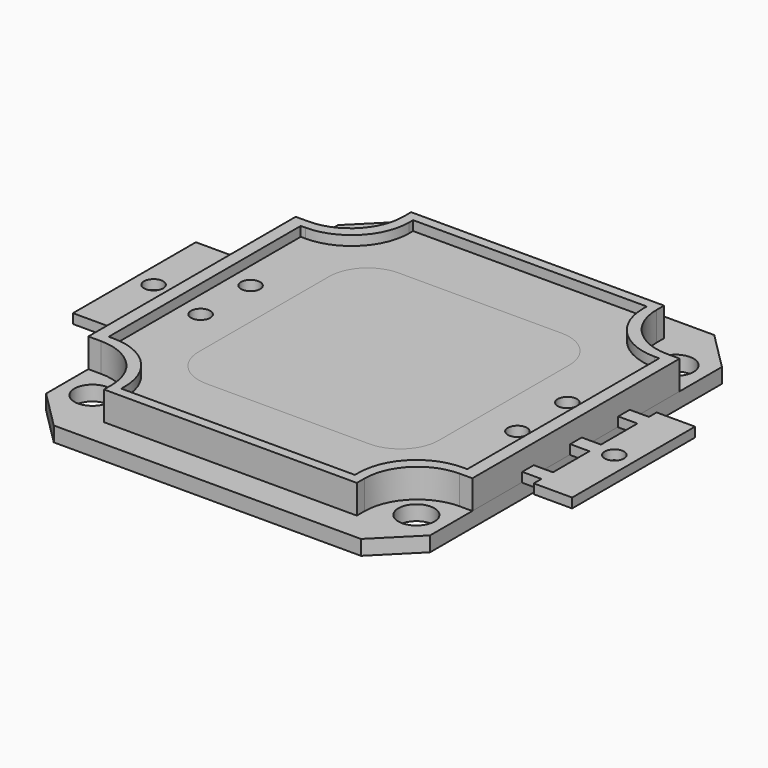
from build123d import *

# Parameters (mm, degrees)
F1_DEPTH = 1.55
F3_SIZE  = 4
F4_R     = 1.875
F5_DEPTH = 4
F6_DEPTH = 3
F2_R     = 1
F2_W     = 1.5
F2_H     = 0.5
F2_W_2   = 0.5
F2_H_2   = 1.5219762474
F2_H_3   = 1.4780237526
F7_DEPTH = 2
F8_DEPTH = 2
F9_START = 1.5
F0_R     = 1
F0_W     = 2
F0_H     = 1.5
F9_DEPTH = 1


with BuildPart() as f1:
    # F0 (on Top) → F1 (new body)
    with BuildSketch(Plane.XY):
        Polygon((20, 23), (-20, 23), (-20, 7), (-20, 5.5), (-20, 0.75), (-20, -0.75), (-20, -5.5), (-20, -7), (-20, -23), (20, -23), (20, -7), (20, -5.5), (20, -0.75), (20, 0.75), (20, 5.5), (20, 7), align=None)
    extrude(amount=F1_DEPTH)

    # F3
    f3_edges = [f1.edges().sort_by_distance(p)[0] for p in [
        (-20, 23, 0.775),
        (20, 23, 0.775),
        (20, -23, 0.775),
        (-20, -23, 0.775),
    ]]
    chamfer(f3_edges, length=F3_SIZE)

    # F4 (on face) → F5 (cut)
    with BuildSketch(Plane.XY.offset(1.55)):
        with Locations((-16.875, -16.875)):
            Circle(F4_R)
        with Locations((16.875, -16.875)):
            Circle(F4_R)
        with Locations((16.875, 16.875)):
            Circle(F4_R)
        with Locations((-16.875, 16.875)):
            Circle(F4_R)
    extrude(amount=-F5_DEPTH, mode=Mode.SUBTRACT)

    # F0 (on Top) → F9 (join)
    with BuildSketch(Plane.XY.offset(F9_START)):
        Polygon((-20, 5.5), (-20, 7), (-22, 7), (-22, 8), (-26, 8), (-26, -8), (-22, -8), (-22, -7), (-20, -7), (-20, -5.5), (-22, -5.5), (-22, -0.75), (-22, 0.75), (-22, 5.5), align=None)
        with Locations((-24, 0)):
            Circle(F0_R, mode=Mode.SUBTRACT)
        Polygon((22, 7), (20, 7), (20, 5.5), (22, 5.5), (22, 0.75), (22, -0.75), (22, -5.5), (20, -5.5), (20, -7), (22, -7), (22, -8), (26, -8), (26, 8), (22, 8), align=None)
        with Locations((24, 0)):
            Circle(F0_R, mode=Mode.SUBTRACT)
        with Locations((21, 0)):
            Rectangle(F0_W, F0_H)
        with Locations((-21, 0)):
            Rectangle(F0_W, F0_H)
    extrude(amount=F9_DEPTH)


with BuildPart() as f6:
    # F2 (on face) → F6 (new body)
    with BuildSketch(Plane.XY.offset(1.55)):
        with BuildLine():
            Line((13.1731458455, 20), (-13.1731458455, 20))
            Line((-13.1731458455, 20), (-13.1731458455, 19))
            ThreePointArc((-13.1731458455, 19), (-14.784058549, 15.1109127035), (-18.6731458455, 13.5))
            Line((-18.6731458455, 13.5), (-20, 13.5))
            Line((-20, 13.5), (-20, -13.5))
            Line((-20, -13.5), (-18.6731458455, -13.5))
            ThreePointArc((-18.6731458455, -13.5), (-14.784058549, -15.1109127035), (-13.1731458455, -19))
            Line((-13.1731458455, -19), (-13.1731458455, -20))
            Line((-13.1731458455, -20), (13.1731458455, -20))
            Line((13.1731458455, -20), (13.1731458455, -19))
            ThreePointArc((13.1731458455, -19), (14.784058549, -15.1109127035), (18.6731458455, -13.5))
            Line((18.6731458455, -13.5), (20, -13.5))
            Line((20, -13.5), (20, 13.5))
            Line((20, 13.5), (18.6731458455, 13.5))
            ThreePointArc((18.6731458455, 13.5), (14.784058549, 15.1109127035), (13.1731458455, 19))
            Line((13.1731458455, 19), (13.1731458455, 20))
        make_face()
        with BuildLine():
            Line((-12.1731458455, 18.5), (-12.1731458455, 19))
            Line((-12.1731458455, 19), (12.1731458455, 19))
            Line((12.1731458455, 19), (12.1731458455, 18.5))
            ThreePointArc((12.1731458455, 18.5), (13.9305051584, 14.2573593129), (18.1731458455, 12.5))
            Line((18.1731458455, 12.5), (18.6731458455, 12.5))
            Line((18.6731458455, 12.5), (18.6731458455, -12.5))
            Line((18.6731458455, -12.5), (18.1731458455, -12.5))
            ThreePointArc((18.1731458455, -12.5), (13.9305051584, -14.2573593129), (12.1731458455, -18.5))
            Line((12.1731458455, -18.5), (12.1731458455, -19))
            Line((12.1731458455, -19), (-12.1731458455, -19))
            Line((-12.1731458455, -19), (-12.1731458455, -18.5))
            ThreePointArc((-12.1731458455, -18.5), (-13.9305051584, -14.2573593129), (-18.1731458455, -12.5))
            Line((-18.1731458455, -12.5), (-18.6731458455, -12.5))
            Line((-18.6731458455, -12.5), (-18.6731458455, 12.5))
            Line((-18.6731458455, 12.5), (-18.1731458455, 12.5))
            ThreePointArc((-18.1731458455, 12.5), (-13.9305051584, 14.2573593129), (-12.1731458455, 18.5))
        make_face(mode=Mode.SUBTRACT)
    extrude(amount=F6_DEPTH)

    # F2 (on face) → F7 (join)
    with BuildSketch(Plane.XY.offset(1.55)):
        with BuildLine():
            Line((12.1731458455, 19), (-12.1731458455, 19))
            Line((-12.1731458455, 19), (-12.1731458455, 18.5))
            ThreePointArc((-12.1731458455, 18.5), (-13.9305051584, 14.2573593129), (-18.1731458455, 12.5))
            Line((-18.1731458455, 12.5), (-18.6731458455, 12.5))
            Line((-18.6731458455, 12.5), (-18.6731458455, -12.5))
            Line((-18.6731458455, -12.5), (-18.1731458455, -12.5))
            ThreePointArc((-18.1731458455, -12.5), (-13.9305051584, -14.2573593129), (-12.1731458455, -18.5))
            Line((-12.1731458455, -18.5), (-12.1731458455, -19))
            Line((-12.1731458455, -19), (12.1731458455, -19))
            Line((12.1731458455, -19), (12.1731458455, -18.5))
            ThreePointArc((12.1731458455, -18.5), (13.9305051584, -14.2573593129), (18.1731458455, -12.5))
            Line((18.1731458455, -12.5), (18.6731458455, -12.5))
            Line((18.6731458455, -12.5), (18.6731458455, 12.5))
            Line((18.6731458455, 12.5), (18.1731458455, 12.5))
            ThreePointArc((18.1731458455, 12.5), (13.9305051584, 14.2573593129), (12.1731458455, 18.5))
            Line((12.1731458455, 18.5), (12.1731458455, 19))
        make_face()
        Polygon((-9.1731458455, -16.4780237526), (-9.1731458455, -18), (-9.6731458455, -18), (-9.6731458455, -16.4780237526), (-11.1731458455, -16.4780237526), (-11.1731458455, -15.9780237526), (-9.6731458455, -15.9780237526), (-9.6731458455, -14.5), (-9.1731458455, -14.5), (-9.1731458455, -15.9780237526), (-7.6731458455, -15.9780237526), (-7.6731458455, -16.4780237526), align=None, mode=Mode.SUBTRACT)
        with Locations((-16.5, -3.25)):
            Circle(F2_R, mode=Mode.SUBTRACT)
        with Locations((16.5, -3.25)):
            Circle(F2_R, mode=Mode.SUBTRACT)
        with Locations((-16.5, 3.25)):
            Circle(F2_R, mode=Mode.SUBTRACT)
        with BuildLine():
            ThreePointArc((-12.5, 8.5), (-11.3284271247, 11.3284271247), (-8.5, 12.5))
            Line((-8.5, 12.5), (8.5, 12.5))
            ThreePointArc((8.5, 12.5), (11.3284271247, 11.3284271247), (12.5, 8.5))
            Line((12.5, 8.5), (12.5, -8.5))
            ThreePointArc((12.5, -8.5), (11.3284271247, -11.3284271247), (8.5, -12.5))
            Line((8.5, -12.5), (-8.5, -12.5))
            ThreePointArc((-8.5, -12.5), (-11.3284271247, -11.3284271247), (-12.5, -8.5))
            Line((-12.5, -8.5), (-12.5, 8.5))
        make_face(mode=Mode.SUBTRACT)
        with Locations((16.5, 3.25)):
            Circle(F2_R, mode=Mode.SUBTRACT)
        with Locations((-8.4231458455, -16.2280237526)):
            Rectangle(F2_W, F2_H)
        with Locations((-10.4231458455, -16.2280237526)):
            Rectangle(F2_W, F2_H)
        with Locations((-9.4231458455, -17.2390118763)):
            Rectangle(F2_W_2, F2_H_2)
        with Locations((-9.4231458455, -15.2390118763)):
            Rectangle(F2_W_2, F2_H_3)
        with Locations((-9.4231458455, -16.2280237526)):
            Rectangle(F2_W_2, F2_H)
    extrude(amount=F7_DEPTH)


with BuildPart() as f8:
    # F2 (on face) → F8 (new body)
    with BuildSketch(Plane.XY.offset(1.55)):
        with BuildLine():
            Line((8.5, 12.5), (-8.5, 12.5))
            ThreePointArc((-8.5, 12.5), (-11.3284271247, 11.3284271247), (-12.5, 8.5))
            Line((-12.5, 8.5), (-12.5, -8.5))
            ThreePointArc((-12.5, -8.5), (-11.3284271247, -11.3284271247), (-8.5, -12.5))
            Line((-8.5, -12.5), (8.5, -12.5))
            ThreePointArc((8.5, -12.5), (11.3284271247, -11.3284271247), (12.5, -8.5))
            Line((12.5, -8.5), (12.5, 8.5))
            ThreePointArc((12.5, 8.5), (11.3284271247, 11.3284271247), (8.5, 12.5))
        make_face()
    extrude(amount=F8_DEPTH)


solid = Compound([f1.part, f6.part, f8.part])
